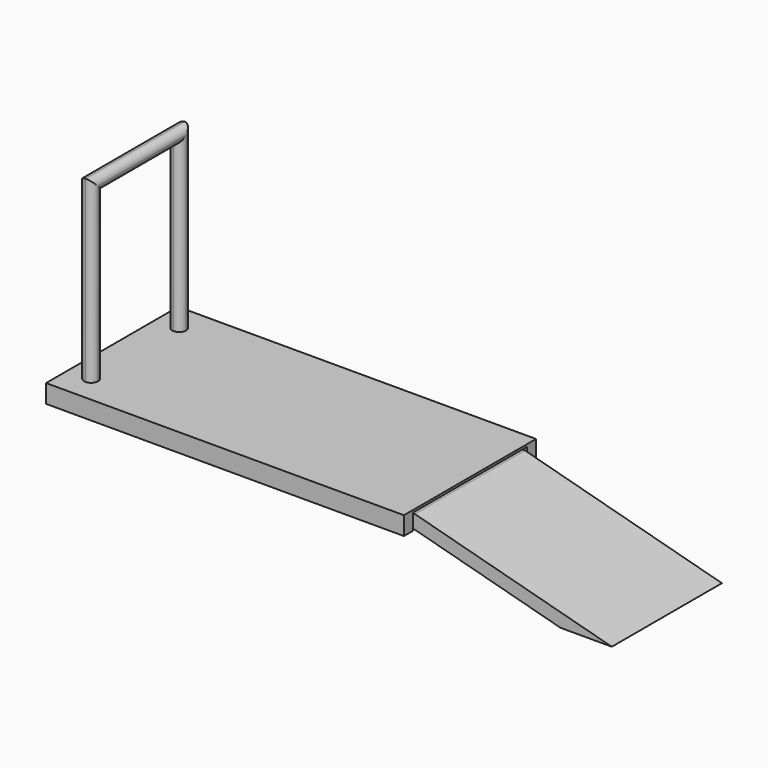
from build123d import *

# Parameters (mm, degrees)
F0_W          = 990.6
F0_H          = 457.2
F1_DEPTH      = 25.4
F1_DEPTH_BACK = 25.4
F2_W          = 38.1
F2_H          = 38.1
F3_DEPTH      = 457.2
F4_W          = 342.9
F4_H          = 38.1
F5_DEPTH      = 38.1
F6_R          = 19.04999
F8_START      = -38.1
F8_DEPTH      = 381
F10_DEPTH     = 228.6
F12_START     = -6.35
F12_DEPTH     = 368.3


# Not quite as in the source:
# - a fillet or chamfer is up to 0.001 mm smaller than in the source, because OpenCascade refuses the exact size


with BuildPart() as f1:
    # F0 (on Top) → F1 (new body, two sides)
    with BuildSketch(Plane.XY) as f1_sk:
        with Locations((495.3, 228.6)):
            Rectangle(F0_W, F0_H)
    extrude(amount=F1_DEPTH)
    extrude(f1_sk.sketch, amount=-F1_DEPTH_BACK)

    # F2 (on face) → F3 (join)
    with BuildSketch(Plane.XY.offset(25.4)):
        with Locations((63.5, 381)):
            Rectangle(F2_W, F2_H)
        with Locations((63.5, 76.2)):
            Rectangle(F2_W, F2_H)
    extrude(amount=F3_DEPTH)

    # F4 (on face) → F5 (join)
    with BuildSketch(Plane(origin=(44.45, 0, 0), x_dir=(0, -1, 0), z_dir=(-1, 0, 0))):
        with Locations((-228.6, 501.65)):
            Rectangle(F4_W, F4_H)
    extrude(amount=-F5_DEPTH)

    # F6 (radius 19.05 in the source; OpenCascade refuses exactly that, so slightly less here)
    f6_edges = [f1.edges().sort_by_distance(p)[0] for p in [
        (82.55, 228.6, 520.7),
        (82.55, 228.6, 482.6),
        (82.55, 361.95, 254),
        (44.45, 361.95, 254),
        (82.55, 400.05, 273.05),
        (82.55, 57.15, 273.05),
        (44.45, 57.15, 273.05),
        (44.45, 228.6, 520.7),
        (44.45, 400.05, 273.05),
        (44.45, 95.25, 254),
        (82.55, 95.25, 254),
        (44.45, 228.6, 482.6),
    ]]
    fillet(f6_edges, radius=F6_R)

    # F7 (on face) → F8 (join)
    with BuildSketch(Plane.XZ.offset(F8_START)):
        Polygon((990.6, -25.4), (1393.4748846771, -133.35), (1535.6660204454, -133.35), (990.6, 12.7), align=None)
    extrude(amount=-F8_DEPTH)

    # F9 (on face) → F10 (cut)
    with BuildSketch(Plane.YZ.offset(990.6)):
        Polygon((425.45, 19.05), (31.75, 19.05), (31.75, -25.4), (38.1, -25.4), (38.1, 12.7), (419.1, 12.7), (419.1, -25.4), (425.45, -25.4), align=None)
    extrude(amount=-F10_DEPTH, mode=Mode.SUBTRACT)

    # F11 (on face) → F12 (cut)
    with BuildSketch(Plane(origin=(0, 419.1, 0), x_dir=(-1, 0, 0), z_dir=(0, 1, 0)).offset(F12_START)):
        Polygon((-990.6, -6.35), (-1464.5704525612, -133.35), (-1393.4748846771, -133.35), (-990.6, -25.4), align=None)
    extrude(amount=-F12_DEPTH, mode=Mode.SUBTRACT)


solid = f1.part
